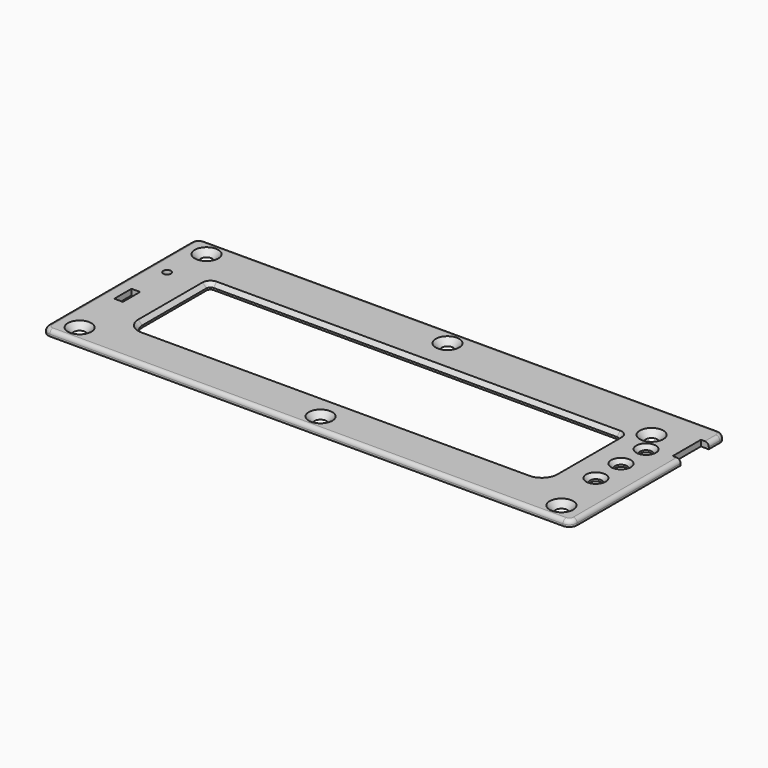
from build123d import *

# Parameters (mm, degrees)
F0_W         = 112.5
F0_H         = 7
F0_R         = 1.5
F0_W_2       = 135
F0_W_3       = 2
F0_H_2       = 2
F0_H_3       = 9
F0_W_4       = 5.5
F0_R_2       = 1
F0_W_5       = 2.2
F0_H_4       = 3.5
F0_H_5       = 9.5
F1_DEPTH     = 1.5
F2_R         = 1
F3_T1_DEPTH  = 6.5
F3_T4_ANGLE  = 90
F3_T6_ANGLE  = 90
F3_T8_ANGLE  = 90
F3_T10_ANGLE = 90
F4_SIZE      = 1
F5_SIZE      = 1
F6_SIZE      = 1.49999


# Not quite as in the source:
# - a fillet or chamfer that OpenCascade refuses, or shapes differently, is made with other operations: its cross-section is extruded or revolved along the edge and cut away or added
# - a fillet or chamfer is up to 0.001 mm smaller than in the source, because OpenCascade refuses the exact size
# - a feature names something its author has since deleted; it is built from what else it names


with BuildPart() as f1:
    # F0 (on Top) → F1 (new body)
    with BuildSketch(Plane.XY):
        Polygon((54.1, 8.075), (54.1, 17.075), (52.1, 17.075), (52.1, 10.075), (-60.4, 10.075), (-60.4, 8.075), (-54.9, 8.075), align=None)
        Polygon((-60.4, 17.075), (52.1, 17.075), (52.1, 19.075), (-62.4, 19.075), (-62.4, 10.075), (-60.4, 10.075), align=None)
        with Locations((-4.15, 13.575)):
            Rectangle(F0_W, F0_H)
        with Locations((-56.4, 14.575)):
            Circle(F0_R, mode=Mode.SUBTRACT)
        with Locations((5.1, 14.575)):
            Circle(F0_R, mode=Mode.SUBTRACT)
        Polygon((54.1, 17.075), (70.6, 17.075), (70.6, 13.575), (72.6, 13.575), (72.6, 19.075), (52.1, 19.075), (52.1, 17.075), align=None)
        Polygon((70.6, 13.575), (70.6, 17.075), (54.1, 17.075), (54.1, 8.075), (-54.9, 8.075), (-54.9, -0.925), (-54.9, -2.925), (-54.9, -21.425), (70.6, -21.425), (70.6, 4.575), align=None)
        with BuildLine():
            Line((56.6, 4.575), (56.6, -15.925))
            ThreePointArc((56.6, -15.925), (55.7213203436, -18.0463203436), (53.6, -18.925))
            Line((53.6, -18.925), (-45.4, -18.925))
            ThreePointArc((-45.4, -18.925), (-47.5213203436, -18.0463203436), (-48.4, -15.925))
            Line((-48.4, -15.925), (-48.4, 4.575))
            ThreePointArc((-48.4, 4.575), (-48.1071067812, 5.2821067812), (-47.4, 5.575))
            Line((-47.4, 5.575), (55.6, 5.575))
            ThreePointArc((55.6, 5.575), (56.3071067812, 5.2821067812), (56.6, 4.575))
        make_face(mode=Mode.SUBTRACT)
        with Locations((64.6, -12.425)):
            Circle(F0_R, mode=Mode.SUBTRACT)
        with Locations((64.6, -4.425)):
            Circle(F0_R, mode=Mode.SUBTRACT)
        with Locations((64.6, 3.575)):
            Circle(F0_R, mode=Mode.SUBTRACT)
        with Locations((61.6, 9.075)):
            Circle(F0_R, mode=Mode.SUBTRACT)
        Polygon((72.6, 4.575), (70.6, 4.575), (70.6, -21.425), (-54.9, -21.425), (-56.55, -21.425), (-58.75, -21.425), (-60.4, -21.425), (-60.4, -2.925), (-62.4, -2.925), (-62.4, -23.425), (72.6, -23.425), align=None)
        with Locations((5.1, -26.925)):
            Rectangle(F0_W_2, F0_H)
        with Locations((-56.4, -25.925)):
            Circle(F0_R, mode=Mode.SUBTRACT)
        with Locations((5.1, -25.925)):
            Circle(F0_R, mode=Mode.SUBTRACT)
        with Locations((66.6, -25.925)):
            Circle(F0_R, mode=Mode.SUBTRACT)
        with Locations((-61.4, 9.075)):
            Rectangle(F0_W_3, F0_H_2)
        with Locations((-61.4, 3.575)):
            Rectangle(F0_W_3, F0_H_3)
        with Locations((-61.4, -1.925)):
            Rectangle(F0_W_3, F0_H_2)
        with Locations((-57.65, 3.575)):
            Rectangle(F0_W_4, F0_H_3)
        with Locations((-57.65, 3.575)):
            Circle(F0_R_2, mode=Mode.SUBTRACT)
        Polygon((-54.9, -2.925), (-54.9, -0.925), (-60.4, -0.925), (-60.4, -2.925), (-58.75, -2.925), (-56.55, -2.925), align=None)
        with Locations((-57.65, -4.675)):
            Rectangle(F0_W_5, F0_H_4)
        Polygon((-56.55, -21.425), (-54.9, -21.425), (-54.9, -2.925), (-56.55, -2.925), (-56.55, -6.425), (-56.55, -11.925), align=None)
        Polygon((-58.75, -2.925), (-60.4, -2.925), (-60.4, -21.425), (-58.75, -21.425), (-58.75, -11.925), (-58.75, -6.425), align=None)
        with Locations((-57.65, -16.675)):
            Rectangle(F0_W_5, F0_H_5)
    extrude(amount=F1_DEPTH)

    # F2
    f2_edges = [f1.edges().sort_by_distance(p)[0] for p in [
        (-62.4, -5.675, 1.5),
        (5.1, 19.075, 1.5),
        (72.6, 16.325, 1.5),
        (72.6, -12.925, 1.5),
        (5.1, -30.425, 1.5),
    ]]
    fillet(f2_edges, radius=F2_R)

    # F3: fillet of radius 2 on 4 edges, made by hand

    # F3_s2 → F3_t1 (cut)
    with BuildSketch(Plane.XY.offset(-5)):
        with BuildLine():
            ThreePointArc((-60.4, 19.075), (-61.8142135624, 18.4892135624), (-62.4, 17.075))
            Line((-62.4, 17.075), (-62.4, 19.075))
            Line((-62.4, 19.075), (-60.4, 19.075))
        make_face()
        with BuildLine():
            ThreePointArc((72.6, 17.075), (72.0142135624, 18.4892135624), (70.6, 19.075))
            Line((70.6, 19.075), (72.6, 19.075))
            Line((72.6, 19.075), (72.6, 17.075))
        make_face()
        with BuildLine():
            ThreePointArc((70.6, -30.425), (72.0142135624, -29.8392135624), (72.6, -28.425))
            Line((72.6, -28.425), (72.6, -30.425))
            Line((72.6, -30.425), (70.6, -30.425))
        make_face()
        with BuildLine():
            ThreePointArc((-62.4, -28.425), (-61.8142135624, -29.8392135624), (-60.4, -30.425))
            Line((-60.4, -30.425), (-62.4, -30.425))
            Line((-62.4, -30.425), (-62.4, -28.425))
        make_face()
    extrude(amount=F3_T1_DEPTH, mode=Mode.SUBTRACT)

    # F3_s3 → F3_t4 (revolve, cut)
    with BuildSketch(Plane.XZ.offset(28.425)):
        with BuildLine():
            ThreePointArc((-61.4, 1.5), (-62.1071067812, 1.2071067812), (-62.4, 0.5))
            Line((-62.4, 0.5), (-62.4, 1.5))
            Line((-62.4, 1.5), (-61.4, 1.5))
        make_face()
    revolve(axis=Axis((-60.4, -28.425, 1.5), (0, 0, 1)), revolution_arc=F3_T4_ANGLE, mode=Mode.SUBTRACT)

    # F3_s5 → F3_t6 (revolve, cut)
    with BuildSketch(Plane.YZ.offset(70.6)):
        with BuildLine():
            ThreePointArc((-29.425, 1.5), (-30.1321067812, 1.2071067812), (-30.425, 0.5))
            Line((-30.425, 0.5), (-30.425, 1.5))
            Line((-30.425, 1.5), (-29.425, 1.5))
        make_face()
    revolve(axis=Axis((70.6, -28.425, 1.5), (0, 0, 1)), revolution_arc=F3_T6_ANGLE, mode=Mode.SUBTRACT)

    # F3_s7 → F3_t8 (revolve, cut)
    with BuildSketch(Plane.XZ.offset(-17.075)):
        with BuildLine():
            ThreePointArc((71.6, 1.5), (72.3071067812, 1.2071067812), (72.6, 0.5))
            Line((72.6, 0.5), (72.6, 1.5))
            Line((72.6, 1.5), (71.6, 1.5))
        make_face()
    revolve(axis=Axis((70.6, 17.075, 1.5), (0, 0, 1)), revolution_arc=F3_T8_ANGLE, mode=Mode.SUBTRACT)

    # F3_s9 → F3_t10 (revolve, cut)
    with BuildSketch(Plane.YZ.offset(-60.4)):
        with BuildLine():
            ThreePointArc((18.075, 1.5), (18.7821067812, 1.2071067812), (19.075, 0.5))
            Line((19.075, 0.5), (19.075, 1.5))
            Line((19.075, 1.5), (18.075, 1.5))
        make_face()
    revolve(axis=Axis((-60.4, 17.075, 1.5), (0, 0, 1)), revolution_arc=F3_T10_ANGLE, mode=Mode.SUBTRACT)

    # F4
    f4_edges = [f1.edges().sort_by_distance(p)[0] for p in [
        (4.1, 5.575, 1.5),
        (55.72132, -18.04632, 1.5),
        (56.6, -5.675, 1.5),
        (56.307107, 5.282107, 1.5),
    ]]
    chamfer(f4_edges, length=F4_SIZE)

    # F5
    f5_edges = [f1.edges().sort_by_distance(p)[0] for p in [
        (63.1, 3.575, 1.5),
        (63.1, -4.425, 1.5),
        (63.1, -12.425, 1.5),
    ]]
    chamfer(f5_edges, length=F5_SIZE)

    # F6 (size 1.5 in the source; OpenCascade refuses exactly that, so slightly less here)
    f6_edges = [f1.edges().sort_by_distance(p)[0] for p in [
        (3.6, 14.575, 1.5),
        (60.1, 9.075, 1.5),
        (65.1, -25.925, 1.5),
        (3.6, -25.925, 1.5),
        (-57.9, -25.925, 1.5),
        (-57.9, 14.575, 1.5),
    ]]
    chamfer(f6_edges, length=F6_SIZE)


solid = f1.part
